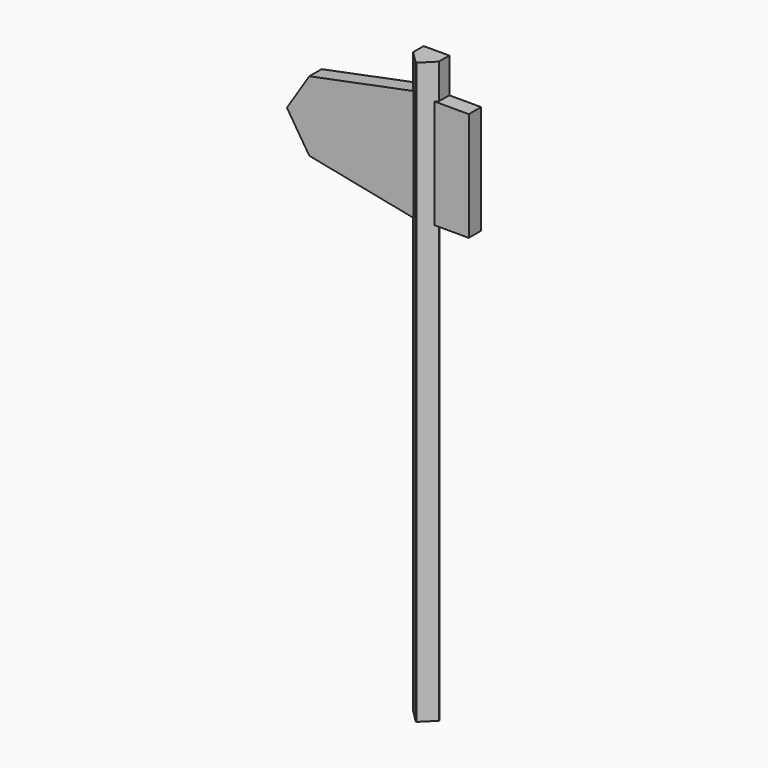
from build123d import *

# Parameters (mm, degrees)
F0_W         = 10.6080286205
F0_H         = 181.0148730874
F1_DEPTH     = 10.52446
F0_W_2       = 13.1920464337
F0_H_2       = 45.1798141003
F2_DEPTH     = 6.38094
F3_T1_DEPTH  = 194.0790226663
F3_T6_DEPTH  = 266.8450713117
F3_T12_DEPTH = 266.8450713117
F3_T18_DEPTH = 266.8450713117
F3_T25_DEPTH = 266.8450713117
F3_T31_DEPTH = 266.8450713117
F3_T37_DEPTH = 266.8450713117
F3_T43_DEPTH = 266.8450713117
F3_T49_DEPTH = 266.8450713117
F3_T56_DEPTH = 266.8450713117
F3_T62_DEPTH = 266.8450713117
F3_T68_DEPTH = 207.1431722451


# Not quite as in the source:
# - a fillet or chamfer that OpenCascade refuses, or shapes differently, is made with other operations: its cross-section is extruded or revolved along the edge and cut away or added


with BuildPart() as f1:
    # F0 (on Front) → F1 (new body)
    with BuildSketch(Plane.XZ):
        with Locations((36.9313266128, -119.8917590082)):
            Rectangle(F0_W, F0_H)
        Polygon((42.2353409231, 15.7954916358), (42.2353409231, 30.3175766021), (31.6273123026, 30.3175766021), (31.6273123026, 16.6022777557), align=None)
        Polygon((42.2353409231, -29.3843224645), (42.2353409231, 15.7954916358), (31.6273123026, 16.6022777557), (31.6273123026, -29.3843224645), align=None)
    extrude(amount=F1_DEPTH)

    # F0 (on Front) → F2 (join)
    with BuildSketch(Plane.XZ):
        Polygon((42.2353409231, 15.7954916358), (42.2353409231, 30.3175766021), (31.6273123026, 30.3175766021), (31.6273123026, 16.6022777557), align=None)
        with Locations((48.8313641399, -6.7944154143)):
            Rectangle(F0_W_2, F0_H_2)
        Polygon((42.2353409231, -29.3843224645), (42.2353409231, 15.7954916358), (31.6273123026, 16.6022777557), (31.6273123026, -29.3843224645), align=None)
        with Locations((36.9313266128, -119.8917590082)):
            Rectangle(F0_W, F0_H)
        Polygon((31.6273123026, -29.3843224645), (31.6273123026, 16.6022777557), (-10.7287643477, 8.1310607493), (-20.0067628175, -6.3910223544), (-10.7287643477, -20.913105458), align=None)
    extrude(amount=F2_DEPTH)

    # F3: chamfer of 5.08 on 4 edges, made by hand

    # F3_s2 → F3_t1 (cut)
    with BuildSketch(Plane.XY.offset(-223.4633451307)):
        Polygon((42.2353409231, -5.08), (37.1553409231, 0), (42.2353409231, 0), align=None)
    extrude(amount=F3_T1_DEPTH, mode=Mode.SUBTRACT)


with BuildPart() as f3_tool4:
    # F3_s5 → F3_t6 (new body)
    with BuildSketch(Plane.XY.offset(-223.4633451307)):
        Polygon((42.2353409231, -5.44446), (37.1553409231, -10.52446), (42.2353409231, -10.52446), align=None)
    extrude(amount=F3_T6_DEPTH)

    split(bisect_by=Plane.XZ.offset(6.38094), keep=Keep.BOTTOM)

    split(bisect_by=Plane.XY.offset(-29.3843224645), keep=Keep.BOTTOM)


with BuildPart() as f1_1:
    add(f1.part)

    # F3_t3: cut F3_tool4
    add(f3_tool4.part, mode=Mode.SUBTRACT)


with BuildPart() as f3_tool10:
    # F3_s11 → F3_t12 (new body)
    with BuildSketch(Plane.XY.offset(-223.4633451307)):
        Polygon((42.2353409231, -5.44446), (37.1553409231, -10.52446), (42.2353409231, -10.52446), align=None)
    extrude(amount=F3_T12_DEPTH)

    split(bisect_by=Plane.XZ.offset(6.38094), keep=Keep.TOP)

    split(bisect_by=Plane.XY.offset(-29.3843224645), keep=Keep.BOTTOM)


with BuildPart() as f1_2:
    add(f1_1.part)

    # F3_t9: cut F3_tool10
    add(f3_tool10.part, mode=Mode.SUBTRACT)


with BuildPart() as f3_tool16:
    # F3_s17 → F3_t18 (new body)
    with BuildSketch(Plane.XY.offset(-223.4633451307)):
        Polygon((42.2353409231, -5.44446), (37.1553409231, -10.52446), (42.2353409231, -10.52446), align=None)
    extrude(amount=F3_T18_DEPTH)

    split(bisect_by=Plane.XY.offset(15.7954916358), keep=Keep.BOTTOM)

    split(bisect_by=Plane.XZ.offset(6.38094), keep=Keep.TOP)

    split(bisect_by=Plane.XY.offset(-29.3843224645), keep=Keep.TOP)


with BuildPart() as f1_3:
    add(f1_2.part)

    # F3_t15: cut F3_tool16
    add(f3_tool16.part, mode=Mode.SUBTRACT)


with BuildPart() as f3_tool23:
    # F3_s24 → F3_t25 (new body)
    with BuildSketch(Plane.XY.offset(-223.4633451307)):
        Polygon((42.2353409231, -5.44446), (37.1553409231, -10.52446), (42.2353409231, -10.52446), align=None)
    extrude(amount=F3_T25_DEPTH)

    split(bisect_by=Plane.XY.offset(15.7954916358), keep=Keep.TOP)

    split(bisect_by=Plane.XZ.offset(6.38094), keep=Keep.BOTTOM)


with BuildPart() as f1_4:
    add(f1_3.part)

    # F3_t22: cut F3_tool23
    add(f3_tool23.part, mode=Mode.SUBTRACT)


with BuildPart() as f3_tool29:
    # F3_s30 → F3_t31 (new body)
    with BuildSketch(Plane.XY.offset(-223.4633451307)):
        Polygon((42.2353409231, -5.44446), (37.1553409231, -10.52446), (42.2353409231, -10.52446), align=None)
    extrude(amount=F3_T31_DEPTH)

    split(bisect_by=Plane.XY.offset(15.7954916358), keep=Keep.TOP)

    split(bisect_by=Plane.XZ.offset(6.38094), keep=Keep.TOP)


with BuildPart() as f1_5:
    add(f1_4.part)

    # F3_t28: cut F3_tool29
    add(f3_tool29.part, mode=Mode.SUBTRACT)


with BuildPart() as f3_tool35:
    # F3_s36 → F3_t37 (new body)
    with BuildSketch(Plane.XY.offset(43.381726181)):
        Polygon((31.6273123026, -5.44446), (36.7073123026, -10.52446), (31.6273123026, -10.52446), align=None)
    extrude(amount=-F3_T37_DEPTH)

    split(bisect_by=Plane.XZ.offset(6.38094), keep=Keep.BOTTOM)

    split(bisect_by=Plane(origin=(-1.976310754, 0, 9.8815518144), x_dir=(0, 1, 0), z_dir=(-0.1961161725, 0, 0.9805806682)), keep=Keep.TOP)


with BuildPart() as f1_6:
    add(f1_5.part)

    # F3_t34: cut F3_tool35
    add(f3_tool35.part, mode=Mode.SUBTRACT)


with BuildPart() as f3_tool41:
    # F3_s42 → F3_t43 (new body)
    with BuildSketch(Plane.XY.offset(43.381726181)):
        Polygon((31.6273123026, -5.44446), (36.7073123026, -10.52446), (31.6273123026, -10.52446), align=None)
    extrude(amount=-F3_T43_DEPTH)

    split(bisect_by=Plane.XZ.offset(6.38094), keep=Keep.TOP)

    split(bisect_by=Plane(origin=(-1.976310754, 0, 9.8815518144), x_dir=(0, 1, 0), z_dir=(-0.1961161725, 0, 0.9805806682)), keep=Keep.TOP)


with BuildPart() as f1_7:
    add(f1_6.part)

    # F3_t40: cut F3_tool41
    add(f3_tool41.part, mode=Mode.SUBTRACT)


with BuildPart() as f3_tool47:
    # F3_s48 → F3_t49 (new body)
    with BuildSketch(Plane.XY.offset(43.381726181)):
        Polygon((31.6273123026, -5.44446), (36.7073123026, -10.52446), (31.6273123026, -10.52446), align=None)
    extrude(amount=-F3_T49_DEPTH)

    split(bisect_by=Plane(origin=(-4.4343967239, 0, -22.1719792319), x_dir=(0, 1, 0), z_dir=(0.1961161725, 0, 0.9805806682)), keep=Keep.TOP)

    split(bisect_by=Plane.XZ.offset(6.38094), keep=Keep.TOP)

    split(bisect_by=Plane(origin=(-1.976310754, 0, 9.8815518144), x_dir=(0, 1, 0), z_dir=(0.1961161725, 0, -0.9805806682)), keep=Keep.TOP)


with BuildPart() as f1_8:
    add(f1_7.part)

    # F3_t46: cut F3_tool47
    add(f3_tool47.part, mode=Mode.SUBTRACT)


with BuildPart() as f3_tool54:
    # F3_s55 → F3_t56 (new body)
    with BuildSketch(Plane.XY.offset(43.381726181)):
        Polygon((31.6273123026, -5.44446), (36.7073123026, -10.52446), (31.6273123026, -10.52446), align=None)
    extrude(amount=-F3_T56_DEPTH)

    split(bisect_by=Plane(origin=(-4.4343967239, 0, -22.1719792319), x_dir=(0, 1, 0), z_dir=(-0.1961161725, 0, -0.9805806682)), keep=Keep.TOP)

    split(bisect_by=Plane.XZ.offset(6.38094), keep=Keep.BOTTOM)


with BuildPart() as f1_9:
    add(f1_8.part)

    # F3_t53: cut F3_tool54
    add(f3_tool54.part, mode=Mode.SUBTRACT)


with BuildPart() as f3_tool60:
    # F3_s61 → F3_t62 (new body)
    with BuildSketch(Plane.XY.offset(43.381726181)):
        Polygon((31.6273123026, -5.44446), (36.7073123026, -10.52446), (31.6273123026, -10.52446), align=None)
    extrude(amount=-F3_T62_DEPTH)

    split(bisect_by=Plane(origin=(-4.4343967239, 0, -22.1719792319), x_dir=(0, 1, 0), z_dir=(-0.1961161725, 0, -0.9805806682)), keep=Keep.TOP)

    split(bisect_by=Plane.XZ.offset(6.38094), keep=Keep.TOP)


with BuildPart() as f1_10:
    add(f1_9.part)

    # F3_t59: cut F3_tool60
    add(f3_tool60.part, mode=Mode.SUBTRACT)


with BuildPart() as f3_tool66:
    # F3_s67 → F3_t68 (new body)
    with BuildSketch(Plane.XY.offset(-16.3201728856)):
        Polygon((31.6273123026, -5.08), (36.7073123026, 0), (31.6273123026, 0), align=None)
    extrude(amount=-F3_T68_DEPTH)

    split(bisect_by=Plane(origin=(-4.4343967239, 0, -22.1719792319), x_dir=(0, 1, 0), z_dir=(-0.1961161725, 0, -0.9805806682)), keep=Keep.TOP)


with BuildPart() as f1_11:
    add(f1_10.part)

    # F3_t65: cut F3_tool66
    add(f3_tool66.part, mode=Mode.SUBTRACT)


solid = f1_11.part
